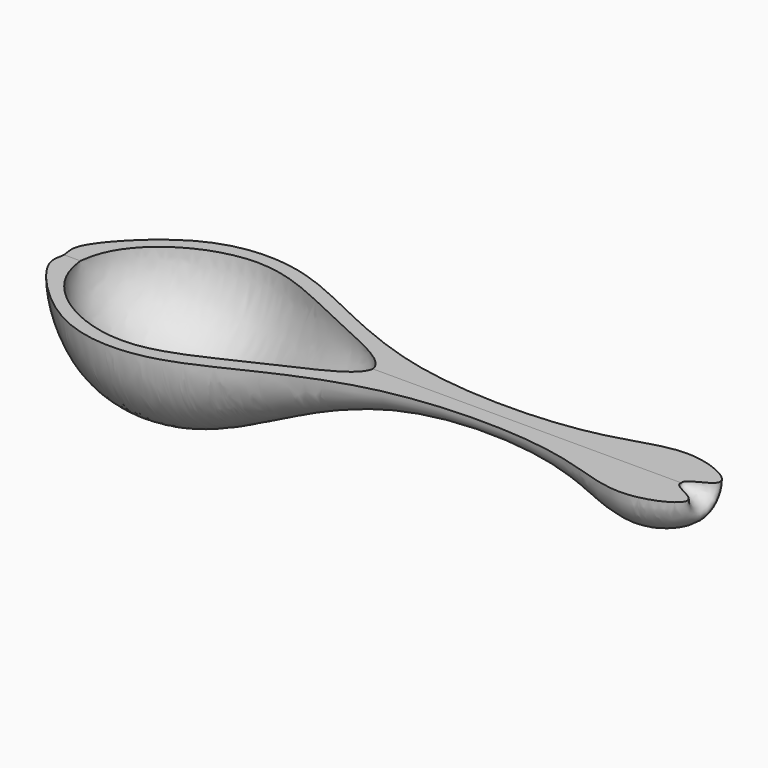
from build123d import *

# Parameters (mm, degrees)
F1_ANGLE = 179.7708248415


with BuildPart() as f1:
    # F0 (on Top) → F1 (revolve)
    with BuildSketch(Plane.XY):
        with BuildLine():
            add(Edge.make_bspline(
                [(-55.6251834087, 0), (-55.780437366, -1.2560242095), (-56.9056941584, -3.882165562), (-44.4254697597, -17.424299561), (-29.874053821, -19.4410469916), (-16.9485259198, -15.2862967849), (6.2641070464, -2.0937167414), (42.0341325096, -2.6263822913), (55.548497101, -10.2721301801), (69.5088780772, -3.3389308093), (60.4579733749, -1.2256101387), (61.0358016439, 0)],
                knots=[0, 0, 0, 0, 0.0553349625, 0.1759761588, 0.2889002074, 0.3951607415, 0.5487827619, 0.724370777, 0.8441010775, 0.9311356719, 1, 1, 1, 1], degree=3))
            Line((61.0358016439, 0), (2.7053091176, 0))
            add(Edge.make_bspline(
                [(-52.5561980903, 0), (-52.3275501625, -1.8695716308), (-51.2915525323, -6.1295654182), (-44.4051598503, -13.470613871), (-29.1159431609, -18.3675095174), (-12.0666682723, -8.6707163034), (2.3721529655, -3.0925535053), (2.7053091176, 0)],
                knots=[0, 0, 0, 0, 0.1359553959, 0.3088168219, 0.5219587702, 0.7784234351, 1, 1, 1, 1], degree=3))
            Line((-52.5561980903, 0), (-55.6251834087, 0))
        make_face()
    revolve(axis=Axis((-54.0906907495, 0, 0), (1, 0, 0)), revolution_arc=F1_ANGLE)


solid = f1.part
